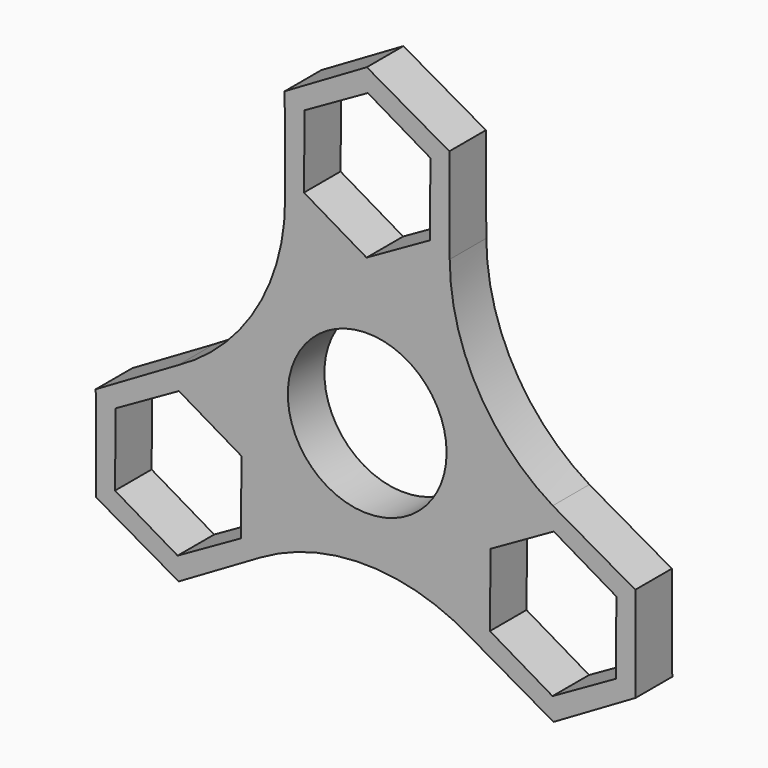
from build123d import *

# Parameters (mm, degrees)
F0_R     = 14.2875
F0_R_2   = 11.0236
F1_DEPTH = 6.35


# Not quite as in the source:
# - a feature names something its author has since deleted; it is built from what else it names


with BuildPart() as f1:
    # F0 (on Front) → F1 (new body)
    with BuildSketch(Plane.XZ):
        with BuildLine():
            ThreePointArc((25.7649177957, -1.6892582355), (15.3069411381, 9.1784817197), (11.4569144183, 23.7611543748))
            Line((11.4569144183, 23.7611543748), (0.05402032, 17.115313105))
            Line((0.05402032, 17.115313105), (-11.4028940983, 23.6675884359))
            ThreePointArc((-11.4028940983, 23.6675884359), (-15.3765179084, 9.0528933251), (-26.2895962669, -1.4487122715))
            Line((-26.2895962669, -1.4487122715), (-14.8326818486, -8.0009876024))
            Line((-14.8326818486, -8.0009876024), (-14.7786615286, -21.1991042031))
            ThreePointArc((-14.7786615286, -21.1991042031), (-0.135152389, -17.3330158123), (14.4160440174, -21.533216106))
            Line((14.4160440174, -21.533216106), (14.3620236974, -8.3350995053))
            Line((14.3620236974, -8.3350995053), (25.7649177957, -1.6892582355))
        make_face()
        Circle(F0_R, mode=Mode.SUBTRACT)
        Circle(F0_R)
        Circle(F0_R_2, mode=Mode.SUBTRACT)
        Polygon((11.4028940983, 36.9592709755), (-0.05402032, 43.5115463064), (-11.4569144183, 36.8657050366), (-11.4028940983, 23.6675884359), (0.05402032, 17.115313105), (11.4569144183, 23.7611543748), align=None)
        Polygon((-8.6923295278, 35.4356960394), (0.089848006, 40.4023410617), (8.7821775338, 35.280074728), (8.6923295278, 25.191163372), (-0.089848006, 20.2245183497), (-8.7821775338, 25.3467846834), align=None, mode=Mode.SUBTRACT)
        Polygon((37.221832214, -8.2415335664), (25.7649177957, -1.6892582355), (14.3620236974, -8.3350995053), (14.4160440174, -21.533216106), (25.8729584357, -28.0854914369), (37.275852534, -21.4396501671), align=None)
        Polygon((17.1266085879, -9.7651085025), (25.9087861217, -4.7984634802), (34.6011156495, -9.9207298139), (34.5112676435, -20.0096411699), (25.7290901097, -24.9762861922), (17.0367605819, -19.8540198585), align=None, mode=Mode.SUBTRACT)
        Polygon((-14.8326818486, -8.0009876024), (-26.2895962669, -1.4487122715), (-37.6924903652, -8.0945535413), (-37.6384700452, -21.292670142), (-26.1815556269, -27.8449454729), (-14.7786615286, -21.1991042031), align=None)
        Polygon((-17.4533984131, -9.6801838499), (-17.5432464191, -19.7690952059), (-26.325423953, -24.7357402282), (-35.0177534808, -19.6134738945), (-34.9279054747, -9.5245625385), (-26.1457279409, -4.5579175162), align=None, mode=Mode.SUBTRACT)
    extrude(amount=F1_DEPTH)


solid = f1.part
